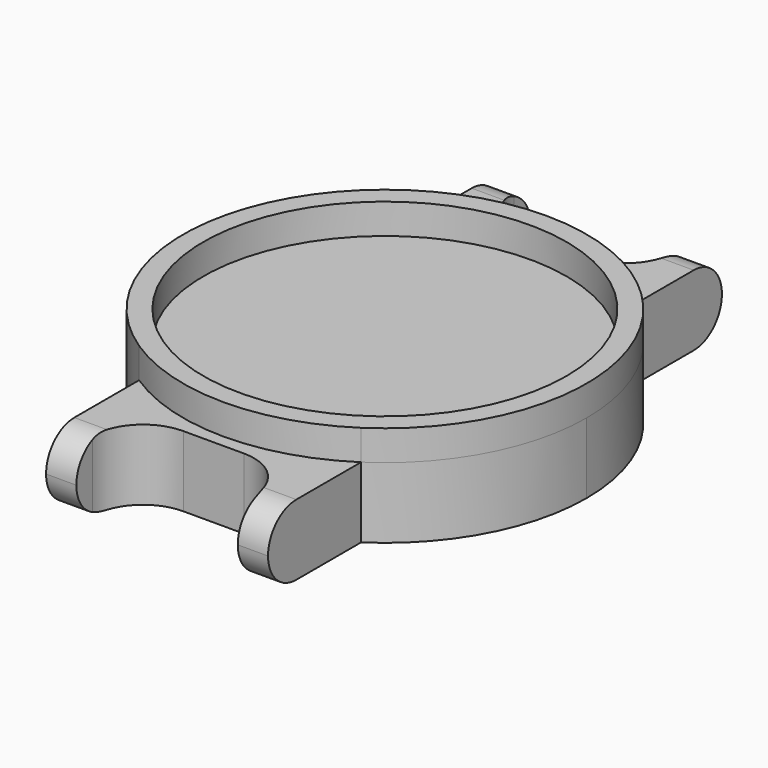
from build123d import *

# Parameters (mm, degrees)
F1_DEPTH = 7
F2_W     = 16
F2_H     = 7
F3_DEPTH = 10
F4_R     = 5
F5_R     = 3.49999
F6_R     = 18
F7_DEPTH = 3


# Not quite as in the source:
# - a fillet or chamfer is up to 0.001 mm smaller than in the source, because OpenCascade refuses the exact size


with BuildPart() as f1:
    # F0 (on Top) → F1 (new body)
    with BuildSketch(Plane.XY):
        with BuildLine():
            ThreePointArc((11, -16.7032930885), (17.6068168617, -9.4868329805), (20, 0))
            ThreePointArc((20, 0), (17.6068168617, 9.4868329805), (11, 16.7032930885))
            Line((11, 16.7032930885), (11, 12))
            Line((11, 12), (-11, 12))
            Line((-11, 12), (-11, 16.7032930885))
            ThreePointArc((-11, 16.7032930885), (-20, 0), (-11, -16.7032930885))
            Line((-11, -16.7032930885), (-11, -11.7698283494))
            Line((-11, -11.7698283494), (11, -11.7698283494))
            Line((11, -11.7698283494), (11, -16.7032930885))
        make_face()
        with BuildLine():
            Line((11, 12), (11, 16.7032930885))
            ThreePointArc((11, 16.7032930885), (0, 20), (-11, 16.7032930885))
            Line((-11, 16.7032930885), (-11, 12))
            Line((-11, 12), (11, 12))
        make_face()
        with BuildLine():
            ThreePointArc((-11, 16.7032930885), (0, 20), (11, 16.7032930885))
            Line((11, 16.7032930885), (11, 28))
            Line((11, 28), (-11, 28))
            Line((-11, 28), (-11, 16.7032930885))
        make_face()
        with BuildLine():
            Line((11, -28.2301716506), (11, -16.7032930885))
            ThreePointArc((11, -16.7032930885), (0, -20), (-11, -16.7032930885))
            Line((-11, -16.7032930885), (-11, -28.2301716506))
            Line((-11, -28.2301716506), (11, -28.2301716506))
        make_face()
        with BuildLine():
            ThreePointArc((-11, -16.7032930885), (0, -20), (11, -16.7032930885))
            Line((11, -16.7032930885), (11, -11.7698283494))
            Line((11, -11.7698283494), (-11, -11.7698283494))
            Line((-11, -11.7698283494), (-11, -16.7032930885))
        make_face()
    extrude(amount=F1_DEPTH)

    # F2 (on face) → F3 (cut)
    with BuildSketch(Plane.XY.offset(7)):
        with Locations((0, 24.5)):
            Rectangle(F2_W, F2_H)
        with Locations((0, -24.7301716506)):
            Rectangle(F2_W, F2_H)
    extrude(amount=-F3_DEPTH, mode=Mode.SUBTRACT)

    # F4
    f4_edges = [f1.edges().sort_by_distance(p)[0] for p in [
        (-8, 21, 3.5),
        (8, 21, 3.5),
        (8, -21.230172, 3.5),
        (-8, -21.230172, 3.5),
    ]]
    fillet(f4_edges, radius=F4_R)

    # F5 (radius 3.5 in the source; OpenCascade refuses exactly that, so slightly less here)
    f5_edges = [f1.edges().sort_by_distance(p)[0] for p in [
        (-9.5, -28.230172, 7),
        (9.5, -28.230172, 7),
        (-9.5, 28, 7),
        (9.5, 28, 7),
        (-9.5, 28, 0),
        (9.5, 28, 0),
        (-9.5, -28.230172, 0),
        (9.5, -28.230172, 0),
    ]]
    fillet(f5_edges, radius=F5_R)

    # F6 (on face) → F7 (join)
    with BuildSketch(Plane.XY.offset(7)):
        with BuildLine():
            Line((11, 16.7032930885), (11, 16.71100699))
            ThreePointArc((11, 16.71100699), (0, 20.0064428277), (-11, 16.71100699))
            Line((-11, 16.71100699), (-11, 16.7032930885))
            ThreePointArc((-11, 16.7032930885), (-20, 0), (-11, -16.7032930885))
            Line((-11, -16.7032930885), (-11, -16.71100699))
            ThreePointArc((-11, -16.71100699), (0, -20.0064428277), (11, -16.71100699))
            Line((11, -16.71100699), (11, -16.7032930885))
            ThreePointArc((11, -16.7032930885), (20, 0), (11, 16.7032930885))
        make_face()
        Circle(F6_R, mode=Mode.SUBTRACT)
    extrude(amount=F7_DEPTH)


solid = f1.part
